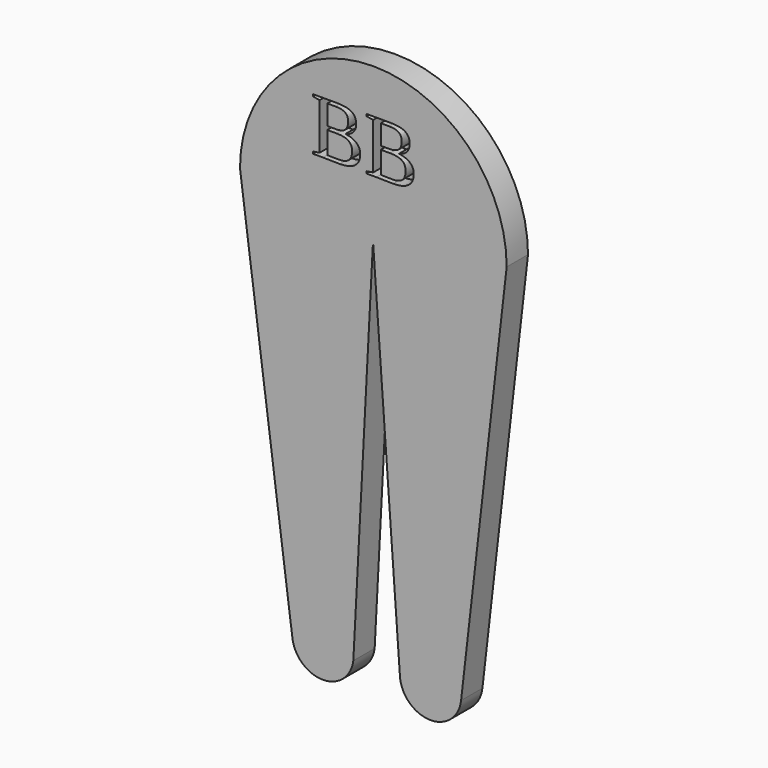
from build123d import *

# Parameters (mm, degrees)
F1_DEPTH     = 2.54
F2_TEXT_SIZE = 7.6401050642
F3_DEPTH     = 1.27


# Not quite as in the source:
# - Text() gives the source's letters only with a copy of the font that has no kerning and outlines rounded to 1/6400 em; it was checked with that copy


with BuildPart() as f1:
    # F0 (on Front) → F1 (new body)
    with BuildSketch(Plane.XZ):
        with BuildLine():
            Line((8.3880713225, -37.7713320923), (12.7302490359, 0))
            ThreePointArc((12.7302490359, 0), (0.0302490359, 12.7), (-12.6697509641, 0))
            Line((-12.6697509641, 0), (-7.6761078074, -37.7713320923))
            ThreePointArc((-7.6761078074, -37.7713320923), (-4.7756311236, -40.3135833392), (-1.8751544397, -37.7713320923))
            Line((-1.8751544397, -37.7713320923), (0, -1.9915634766))
            Line((0, -1.9915634766), (2.5745187556, -37.7713320923))
            ThreePointArc((2.5745187556, -37.7713320923), (5.481295039, -40.363091015), (8.3880713225, -37.7713320923))
        make_face()
    extrude(amount=F1_DEPTH)

    # F2 (on face) → F3 (cut)
    with BuildSketch(Plane.XZ.offset(2.54)):
        with Locations((-5.9401025064, 3.4826842602)):
            Text('BB', F2_TEXT_SIZE, font='Tinos', text_align=(TextAlign.LEFT, TextAlign.BOTTOM))
    extrude(amount=-F3_DEPTH, mode=Mode.SUBTRACT)


solid = f1.part
